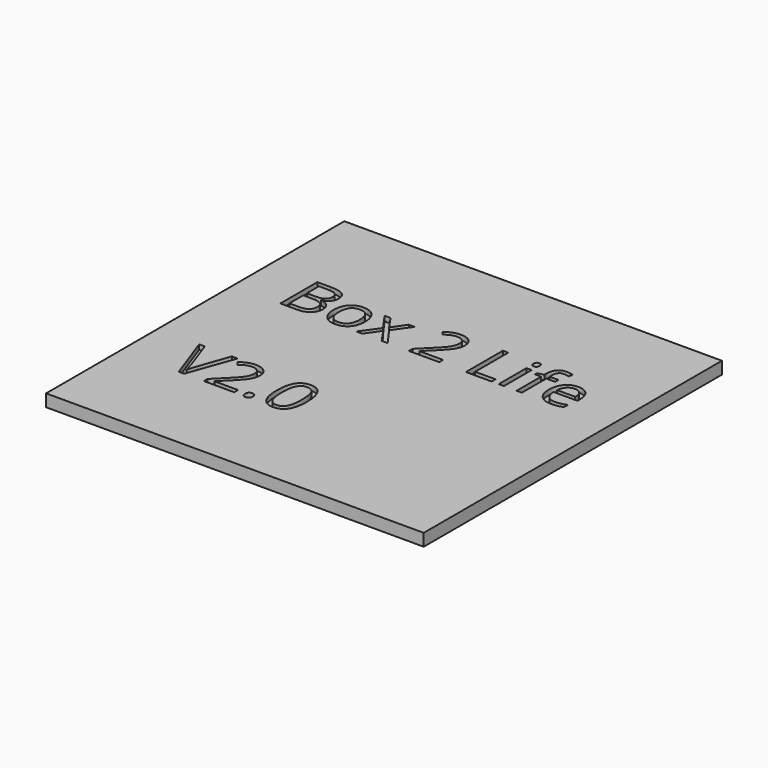
from build123d import *

# Parameters (mm, degrees)
F0_W         = 77
F0_H         = 76
F1_DEPTH     = 2.5
F2_TEXT_SIZE = 13.1944444444
F3_DEPTH     = 1


# Not quite as in the source:
# - Text() gives the source's letters only with a copy of the font that has no kerning and outlines rounded to 1/6400 em; it was checked with that copy


with BuildPart() as f1:
    # F0 (on Top) → F1 (new body)
    with BuildSketch(Plane.XY):
        with Locations((38.5, 38)):
            Rectangle(F0_W, F0_H)
    extrude(amount=F1_DEPTH)

    # F2 (on face) → F3 (cut)
    with BuildSketch(Plane.XY.offset(2.5)):
        with Locations((8.4702690972, 47.5)):
            Text('Box 2 Life', F2_TEXT_SIZE, font='Open Sans', text_align=(TextAlign.LEFT, TextAlign.BOTTOM))
        with Locations((8.4702690972, 19)):
            Text('V2.0', F2_TEXT_SIZE, font='Open Sans', text_align=(TextAlign.LEFT, TextAlign.BOTTOM))
    extrude(amount=-F3_DEPTH, mode=Mode.SUBTRACT)


solid = f1.part
